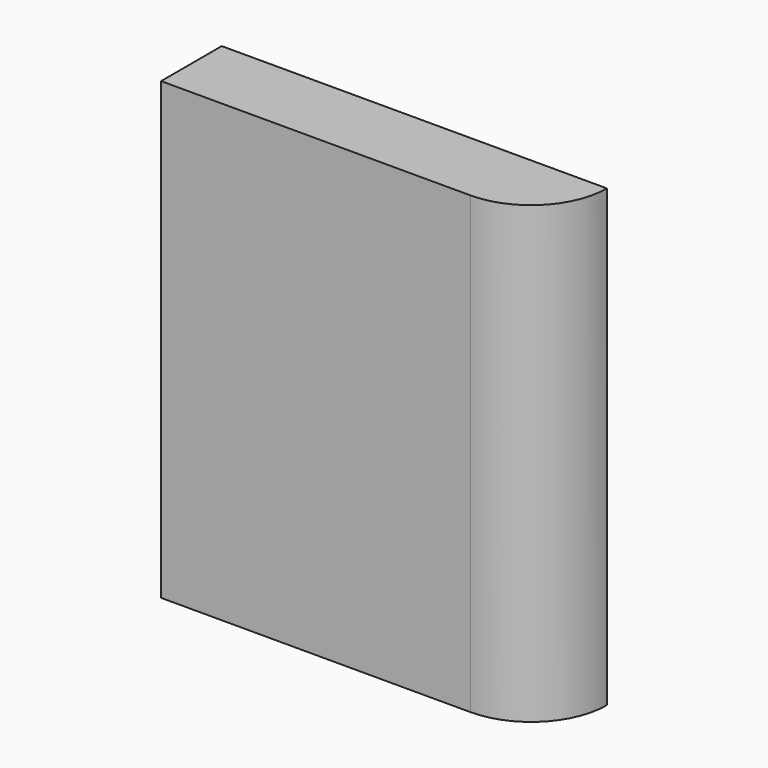
from build123d import *

# Parameters (mm, degrees)
F0_W     = 254
F0_H     = 300
F2_DEPTH = 50
F3_R     = 49.99999


# Not quite as in the source:
# - a fillet or chamfer is up to 0.001 mm smaller than in the source, because OpenCascade refuses the exact size


with BuildPart() as f2:
    # F0 (on Front) → F2 (new body)
    with BuildSketch(Plane.XZ):
        Rectangle(F0_W, F0_H)
    extrude(amount=F2_DEPTH)

    # F3 (radius 50 in the source; OpenCascade refuses exactly that, so slightly less here)
    f3_edges = [f2.edges().sort_by_distance(p)[0] for p in [
        (127, -50, 0),
    ]]
    fillet(f3_edges, radius=F3_R)


solid = f2.part
